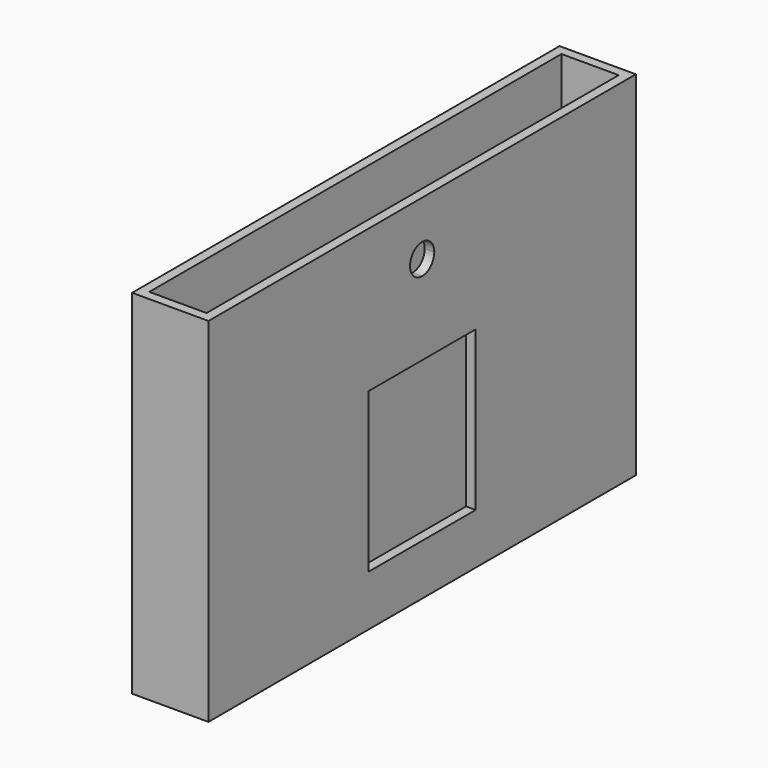
from build123d import *

# Parameters (mm, degrees)
F0_W     = 152.4
F0_H     = 1066.8
F0_W_2   = 114.3
F0_H_2   = 1028.7
F1_DEPTH = 704.85
F3_DEPTH = 25.4
F5_DEPTH = 25.4


# Not quite as in the source:
# - a feature names something its author has since deleted; it is built from what else it names


with BuildPart() as f1:
    # F0 (on Top) → F1 (new body)
    with BuildSketch(Plane.XY):
        Rectangle(F0_W, F0_H)
        Rectangle(F0_W_2, F0_H_2, mode=Mode.SUBTRACT)
    extrude(amount=F1_DEPTH)

    # F2 (on face) → F3 (cut)
    with BuildSketch(Plane.YZ.offset(76.2)):
        with BuildLine():
            ThreePointArc((30.226, 596.9), (-21.3730095681, 618.2730095681), (0, 566.674))
            ThreePointArc((0, 566.674), (21.3730095681, 575.5269904319), (30.226, 596.9))
        make_face()
        Polygon((-133.35, 101.6), (0, 101.6), (133.35, 101.6), (133.35, 419.1), (0, 419.1), (-133.35, 419.1), align=None)
    extrude(amount=-F3_DEPTH, mode=Mode.SUBTRACT)

    # F4 (on face) → F5 (cut)
    with BuildSketch(Plane(origin=(-76.2, 0, 0), x_dir=(0, -1, 0), z_dir=(-1, 0, 0))):
        with BuildLine():
            ThreePointArc((30.226, 406.4), (-21.3730095681, 427.7730095681), (0, 376.174))
            ThreePointArc((0, 376.174), (21.3730095681, 385.0269904319), (30.226, 406.4))
        make_face()
    extrude(amount=-F5_DEPTH, mode=Mode.SUBTRACT)


solid = f1.part
